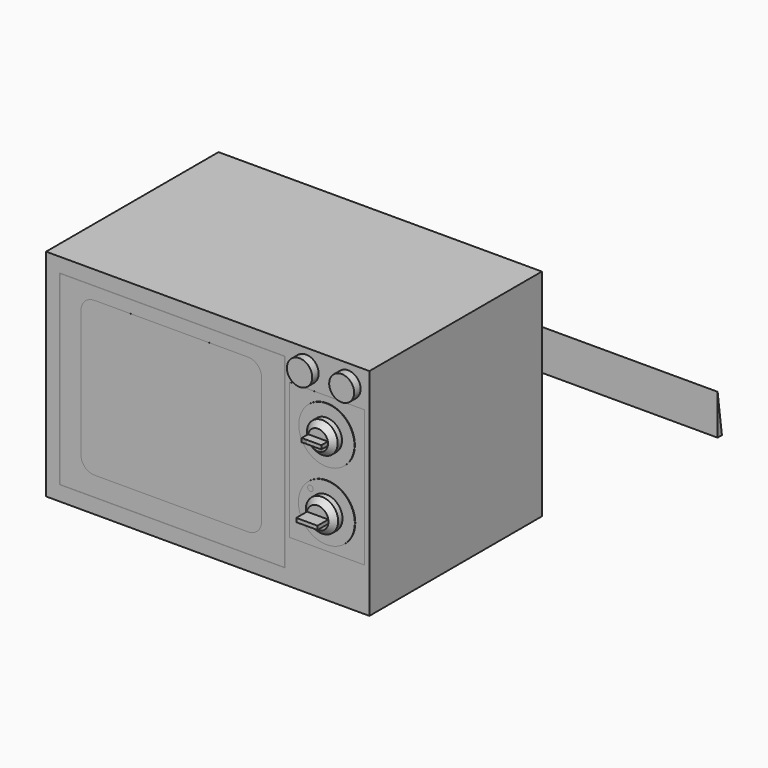
from build123d import *

# Parameters (mm, degrees)
F0_W        = 600
F0_H        = 400
F1_DEPTH    = 400
F3_W        = 418.2137697935
F3_H        = 345.9964096546
F4_DEPTH    = 0.01
F5_T1_DEPTH = 349.5315899895
F5_T3_DEPTH = 421.7489501284
F7_DEPTH    = 0.01
F8_R        = 23.4792892743
F9_DEPTH    = 15
F8_R_2      = 23.149137583
F10_W       = 138.5136842728
F10_H       = 253.5866200924
F11_DEPTH   = 0.01
F12_R       = 51.6479650584
F13_DEPTH   = 1
F12_R_2     = 52.4009870451
F14_R       = 28.5626068182
F15_DEPTH   = 20
F14_R_2     = 30.0445594594
F16_SIZE    = 10
F16_2_SIZE  = 10
F17_W       = 36.4593127685
F17_H       = 7
F18_DEPTH   = 15
F19_W       = 39.4732498749
F19_H       = 7
F20_DEPTH   = 25
F21_W       = 450
F21_H       = 300
F22_DEPTH   = 15
F23_R       = 5.1925071587
F24_DEPTH   = 0.01
F26_DEPTH   = 0.01
F28_DEPTH   = 600


# Not quite as in the source:
# - a fillet or chamfer that OpenCascade refuses, or shapes differently, is made with other operations: its cross-section is extruded or revolved along the edge and cut away or added
# - a feature names something its author has since deleted; it is built from what else it names


with BuildPart() as f1:
    # F0 (on Front) → F1 (new body)
    with BuildSketch(Plane.XZ):
        with Locations((0.952295959, -5.4897558531)):
            Rectangle(F0_W, F0_H)
    extrude(amount=F1_DEPTH)


with BuildPart() as f4:
    # F3 (on face) → F4 (new body)
    with BuildSketch(Plane.XZ.offset(400)):
        with Locations((-65.1162043214, -5.0687789917)):
            Rectangle(F3_W, F3_H)
    extrude(amount=F4_DEPTH)

    # F5: fillet of radius 25 on 4 edges, made by hand

    # F5_s2 → F5_t1 (cut)
    with BuildSketch(Plane.XY.offset(-179.8345739864)):
        with BuildLine():
            ThreePointArc((143.9906805754, -400), (143.637197899, -400.007499875), (143.2836445084, -400.01))
            Line((143.2836445084, -400.01), (143.9906805754, -400.01))
            Line((143.9906805754, -400.01), (143.9906805754, -400))
        make_face()
        with BuildLine():
            ThreePointArc((-274.2230892181, -400), (-273.8696065418, -400.007499875), (-273.5160531512, -400.01))
            Line((-273.5160531512, -400.01), (-274.2230892181, -400.01))
            Line((-274.2230892181, -400.01), (-274.2230892181, -400))
        make_face()
    extrude(amount=F5_T1_DEPTH, mode=Mode.SUBTRACT)

    # F5_s4 → F5_t3 (cut)
    with BuildSketch(Plane.YZ.offset(-275.9906793856)):
        with BuildLine():
            ThreePointArc((-400, 167.9294258356), (-400.007499875, 167.5759431592), (-400.01, 167.2223897686))
            Line((-400.01, 167.2223897686), (-400.01, 167.9294258356))
            Line((-400.01, 167.9294258356), (-400, 167.9294258356))
        make_face()
        with BuildLine():
            ThreePointArc((-400, -178.066983819), (-400.007499875, -177.7135011426), (-400.01, -177.359947752))
            Line((-400.01, -177.359947752), (-400.01, -178.066983819))
            Line((-400.01, -178.066983819), (-400, -178.066983819))
        make_face()
    extrude(amount=F5_T3_DEPTH, mode=Mode.SUBTRACT)


with BuildPart() as f7:
    # F6 (on face) → F7 (new body)
    with BuildSketch(Plane.XZ.offset(400.01)):
        with BuildLine():
            Line((75.8758544922, 144.1260868311), (-209.3418747187, 144.1260868311))
            ThreePointArc((-209.3418747187, 144.1260868311), (-227.0195442483, 136.8037563608), (-234.3418747187, 119.1260868311))
            Line((-234.3418747187, 119.1260868311), (-234.3418747187, -116.4193958044))
            ThreePointArc((-234.3418747187, -116.4193958044), (-227.0195442483, -134.0970653341), (-209.3418747187, -141.4193958044))
            Line((-209.3418747187, -141.4193958044), (75.8758544922, -141.4193958044))
            ThreePointArc((75.8758544922, -141.4193958044), (93.5535240219, -134.0970653341), (100.8758544922, -116.4193958044))
            Line((100.8758544922, -116.4193958044), (100.8758544922, 119.1260868311))
            ThreePointArc((100.8758544922, 119.1260868311), (93.5535240219, 136.8037563608), (75.8758544922, 144.1260868311))
        make_face()
    extrude(amount=F7_DEPTH)


with BuildPart() as f9:
    # F8 (on face) → F9 (new body)
    with BuildSketch(Plane.XZ.offset(400)):
        with Locations((183.3329312503, 159.8454117775)):
            Circle(F8_R)
    extrude(amount=F9_DEPTH)


with BuildPart() as f9b:
    # F8 (on face) → F9, piece 2 (new body)
    with BuildSketch(Plane.XZ.offset(400)):
        with Locations((261.4785395563, 159.8454117775)):
            Circle(F8_R_2)
    extrude(amount=F9_DEPTH)


with BuildPart() as f11:
    # F10 (on face) → F11 (new body)
    with BuildSketch(Plane.XZ.offset(400)):
        with Locations((222.3730683327, 1.4600753784)):
            Rectangle(F10_W, F10_H)
    extrude(amount=F11_DEPTH)


with BuildPart() as f13:
    # F12 (on face) → F13 (new body)
    with BuildSketch(Plane.XZ.offset(400.01)):
        with Locations((222.3730683327, 64.8567304015)):
            Circle(F12_R)
    extrude(amount=F13_DEPTH)


with BuildPart() as f13b:
    # F12 (on face) → F13, piece 2 (new body)
    with BuildSketch(Plane.XZ.offset(400.01)):
        with Locations((222.3730683327, -61.9365796447)):
            Circle(F12_R_2)
    extrude(amount=F13_DEPTH)


with BuildPart() as f15:
    # F14 (on face) → F15 (new body)
    with BuildSketch(Plane.XZ.offset(401.01)):
        with Locations((222.3730683327, 64.8567304015)):
            Circle(F14_R)
    extrude(amount=F15_DEPTH)

    # F16
    f16_edges = [f15.edges().sort_by_distance(p)[0] for p in [
        (193.810462, -421.01, 64.85673),
    ]]
    chamfer(f16_edges, length=F16_SIZE)


with BuildPart() as f15b:
    # F14 (on face) → F15, piece 2 (new body)
    with BuildSketch(Plane.XZ.offset(401.01)):
        with Locations((221.7598557472, -62.2995458543)):
            Circle(F14_R_2)
    extrude(amount=F15_DEPTH)

    # F16#2
    f16_2_edges = [f15b.edges().sort_by_distance(p)[0] for p in [
        (191.715296, -421.01, -62.299546),
    ]]
    chamfer(f16_2_edges, length=F16_2_SIZE)

    # F19 (on face) → F20 (join)
    with BuildSketch(Plane.XZ.offset(421.01)):
        with Locations((221.7598557472, -62.2995458543)):
            Rectangle(F19_W, F19_H)
    extrude(amount=F20_DEPTH)


with BuildPart() as f18:
    # F17 (on face) → F18 (new body)
    with BuildSketch(Plane.XZ.offset(421.01)):
        with Locations((222.3730683327, 64.8567304015)):
            Rectangle(F17_W, F17_H)
    extrude(amount=F18_DEPTH)


with BuildPart() as f22:
    # F21 (on face) → F22 (new body)
    with BuildSketch(Plane(origin=(0, 0, -205.4897558531), x_dir=(1, 0, 0), z_dir=(0, 0, -1))):
        with Locations((0, 195.795734788)):
            Rectangle(F21_W, F21_H)
    extrude(amount=F22_DEPTH)


with BuildPart() as f24:
    # F23 (on face) → F24 (new body)
    with BuildSketch(Plane.XZ.offset(401.01)):
        with Locations((192.378346444, -31.941857756)):
            Circle(F23_R)
    extrude(amount=F24_DEPTH)


with BuildPart() as f26:
    # F25 (on face) → F26 (new body)
    with BuildSketch(Plane.XZ.offset(436.01)):
        Polygon((213.2582401405, 63.1067304015), (213.2582401405, 66.6067304015), (206.0518860817, 64.8567304015), align=None)
    extrude(amount=F26_DEPTH)


with BuildPart() as f28:
    # F27 (on Right) → F28 (new body)
    with BuildSketch(Plane.YZ):
        Polygon((43.9466453344, 6.5159001984), (33.9466453344, 81.5159001984), (33.9466453344, 6.5159001984), align=None)
    extrude(amount=F28_DEPTH)


solid = Compound([f1.part, f4.part, f7.part, f9.part, f9b.part, f11.part, f13.part, f13b.part, f15.part, f15b.part, f18.part, f22.part, f24.part, f26.part, f28.part])
